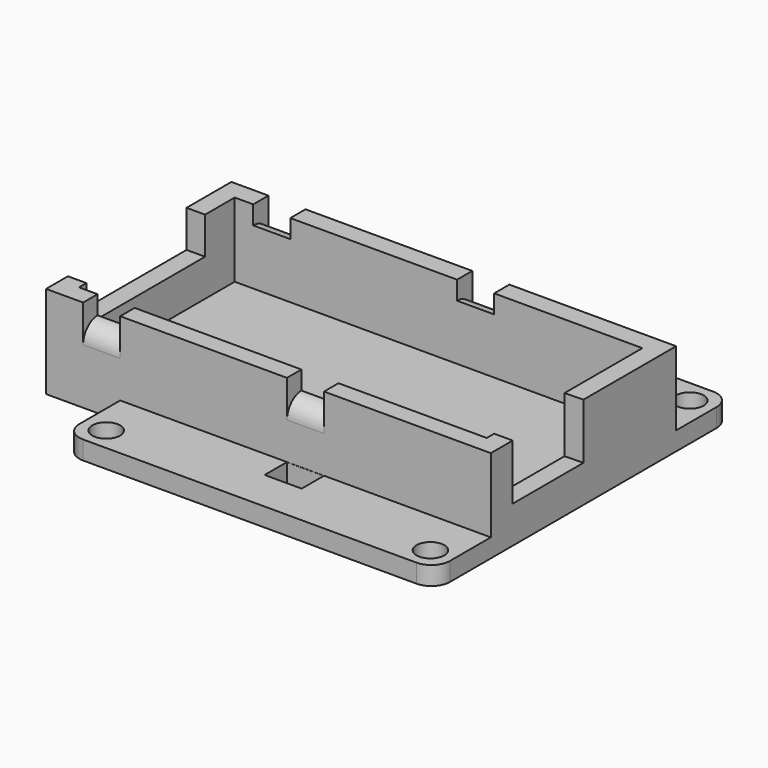
from build123d import *

# Parameters (mm, degrees)
F1_DEPTH     = 2
F2_R         = 2
F3_D         = 3
F7_DEPTH     = 2
F6_W         = 4
F6_H         = 1.95
F6_H_2       = 2.05
F6_H_3       = 2.0331665652
F8_DEPTH     = 8
F6_W_2       = 18
F9_DEPTH     = 10
F10_T1_DEPTH = 4
F10_T3_DEPTH = 4
F11_DEPTH    = 4
F6_W_3       = 2
F6_H_4       = 16
F12_DEPTH    = 6


# Not quite as in the source:
# - a fillet or chamfer that OpenCascade refuses, or shapes differently, is made with other operations: its cross-section is extruded or revolved along the edge and cut away or added


with BuildPart() as f1:
    # F0 (on Top) → F1 (new body)
    with BuildSketch(Plane.XY):
        Polygon((-19.8978664808, -19.9668334348), (0.1021335192, -19.9668334348), (0.1021335192, -15.4668334348), (-1.8978664808, -15.4668334348), (-1.8978664808, -12.4668334348), (0.1021335192, -12.4668334348), (0.1021335192, 0.0331665652), (-19.8978664808, 0.0331665652), align=None)
    extrude(amount=F1_DEPTH)

    # F2
    f2_edges = [f1.edges().sort_by_distance(p)[0] for p in [
        (-19.897866, -19.966833, 1),
    ]]
    fillet(f2_edges, radius=F2_R)

    # F3 (through all)
    with Locations(Plane(origin=(0, 0, 0), x_dir=(1, 0, 0), z_dir=(0, 0, -1))):
        with Locations((-17.3978664808, 17.4668334348)):
            Hole(F3_D / 2)

    # F4: F1 across face


with BuildPart() as f1_1:
    add(f1.part)
    add(f1.part.mirror(Plane(origin=(0.1021335192, -6.2168334348, 1), x_dir=(0, 1, 0), z_dir=(1, 0, 0))))

    # F5: F1 across face


with BuildPart() as f1_2:
    add(f1_1.part)
    add(f1_1.part.mirror(Plane(origin=(0.1021335192, 0.0331665652, 1), x_dir=(-1, 0, 0), z_dir=(0, 1, 0))))

    # F6 (on face) → F7 (join)
    with BuildSketch(Plane(origin=(0, 0, 0), x_dir=(1, 0, 0), z_dir=(0, 0, -1))):
        Polygon((-25.8978664808, -10.5), (-23.8978664808, -10.5), (-19.8978664808, -10.5), (-19.8978664808, 10.5), (-23.8978664808, 10.5), (-25.8978664808, 10.5), (-25.8978664808, 9.5), (-25.8978664808, -6.5), align=None)
        Polygon((18.1021335192, 0), (20.1021335192, -0.05), (20.1021335192, 9.5), (18.1021335192, 9.5), align=None)
        Polygon((-19.8978664808, 10.5), (-19.8978664808, -10.5), (-1.8978664808, -10.5), (2.1021335192, -10.5), (18.1021335192, -10.5), (18.1021335192, 0), (18.1021335192, 9.5), (18.1021335192, 10.5), (2.1021335192, 10.5), (-1.8978664808, 10.5), align=None)
    extrude(amount=-F7_DEPTH)

    # F6 (on face) → F8 (join)
    with BuildSketch(Plane(origin=(0, 0, 0), x_dir=(1, 0, 0), z_dir=(0, 0, -1))):
        with Locations((-21.8978664808, 11.475)):
            Rectangle(F6_W, F6_H)
        with Locations((-21.8978664808, -11.525)):
            Rectangle(F6_W, F6_H_2)
        with Locations((0.1021335192, -11.5165832826)):
            Rectangle(F6_W, F6_H_3)
        with Locations((0.1021335192, 11.475)):
            Rectangle(F6_W, F6_H)
    extrude(amount=-F8_DEPTH)

    # F6 (on face) → F9 (join)
    with BuildSketch(Plane(origin=(0, 0, 0), x_dir=(1, 0, 0), z_dir=(0, 0, -1))):
        Polygon((-27.8978664808, -12.55), (-23.8978664808, -12.55), (-23.8978664808, -10.5), (-25.8978664808, -10.5), (-25.8978664808, -6.5), (-27.8978664808, -6.5), align=None)
        Polygon((-27.8978664808, 12.45), (-27.8978664808, 9.5), (-25.8978664808, 9.5), (-25.8978664808, 10.5), (-23.8978664808, 10.5), (-23.8978664808, 12.45), align=None)
        Polygon((-19.8978664808, -10.5), (-19.8978664808, -12.55), (-1.8978664808, -12.55), (-1.8978664808, -12.5331665652), (-1.8978664808, -10.5), align=None)
        Polygon((2.1021335192, -12.5331665652), (2.1021335192, -12.55), (20.1021335192, -12.55), (20.1021335192, -0.05), (18.1021335192, 0), (18.1021335192, -10.5), (2.1021335192, -10.5), align=None)
        Polygon((2.1021335192, 12.45), (2.1021335192, 10.5), (18.1021335192, 10.5), (18.1021335192, 9.5), (20.1021335192, 9.5), (20.1021335192, 12.45), align=None)
        with Locations((-10.8978664808, 11.475)):
            Rectangle(F6_W_2, F6_H)
    extrude(amount=-F9_DEPTH)

    # F10: fillet of radius 2 on 4 edges, made by hand

    # F10_s2 → F10_t1 (cut)
    with BuildSketch(Plane.YZ.offset(-23.8978664808)):
        with BuildLine():
            ThreePointArc((10.55, 8), (11.9642135624, 7.4142135624), (12.55, 6))
            Line((12.55, 6), (12.55, 8))
            Line((12.55, 8), (10.55, 8))
        make_face()
        with BuildLine():
            ThreePointArc((-12.45, 6), (-11.8642135624, 7.4142135624), (-10.45, 8))
            Line((-10.45, 8), (-12.45, 8))
            Line((-12.45, 8), (-12.45, 6))
        make_face()
    extrude(amount=F10_T1_DEPTH, mode=Mode.SUBTRACT)

    # F10_s4 → F10_t3 (cut)
    with BuildSketch(Plane.YZ.offset(-1.8978664808)):
        with BuildLine():
            ThreePointArc((-12.45, 6), (-11.8642135624, 7.4142135624), (-10.45, 8))
            Line((-10.45, 8), (-12.45, 8))
            Line((-12.45, 8), (-12.45, 6))
        make_face()
        with BuildLine():
            ThreePointArc((12.5331665652, 6), (11.9473801276, 7.4142135624), (10.5331665652, 8))
            Line((10.5331665652, 8), (12.5331665652, 8))
            Line((12.5331665652, 8), (12.5331665652, 6))
        make_face()
    extrude(amount=F10_T3_DEPTH, mode=Mode.SUBTRACT)

    # F6 (on face) → F11 (join)
    with BuildSketch(Plane(origin=(0, 0, 0), x_dir=(1, 0, 0), z_dir=(0, 0, -1))):
        Polygon((18.1021335192, 0), (20.1021335192, -0.05), (20.1021335192, 9.5), (18.1021335192, 9.5), align=None)
    extrude(amount=-F11_DEPTH)

    # F6 (on face) → F12 (join)
    with BuildSketch(Plane(origin=(0, 0, 0), x_dir=(1, 0, 0), z_dir=(0, 0, -1))):
        with Locations((-26.8978664808, 1.5)):
            Rectangle(F6_W_3, F6_H_4)
    extrude(amount=-F12_DEPTH)


solid = f1_2.part
